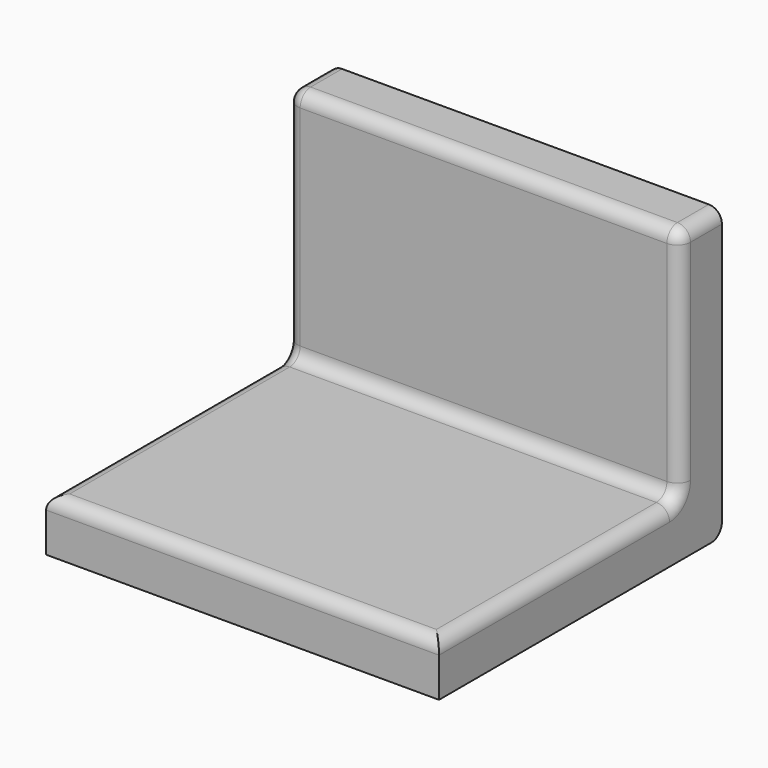
from build123d import *

# Parameters (mm, degrees)
F0_W    = 300
F0_H    = 40
F3_F1_R = 10
F3_F2_R = 10


with BuildPart() as f2:
    # F2: sweep along a path in F1
    with BuildLine(Plane.YZ) as f2_path:
        Line((0, 0), (250, 0))
        Line((250, 0), (250, 200))
    # F0 (on Front) → F2 (sweep)
    with BuildSketch(Plane.XZ):
        with Locations((4.6769320033, 0)):
            Rectangle(F0_W, F0_H)
    sweep(path=f2_path.line, transition=Transition.RIGHT)

    # F3: fillet of radius 10 on 8 edges, made by hand

    # F3_f1
    f3_f1_edges = [f2.edges().sort_by_distance(p)[0] for p in [
        (4.6769320033, 230, 20),
    ]]
    fillet(f3_f1_edges, radius=F3_F1_R)

    # F3_f2
    f3_f2_edges = [f2.edges().sort_by_distance(p)[0] for p in [
        (154.6769320033, 250, 200),
        (-145.3230679967, 250, 200),
        (154.6769320033, 110, 20),
        (4.6769320033, 0, 20),
        (-145.3230679967, 110, 20),
        (4.6769320033, 270, -20),
        (4.6769320033, 230, 200),
        (-145.3230679967, 227.0710678119, 22.9289321881),
        (154.6769320033, 227.0710678119, 22.9289321881),
    ]]
    fillet(f3_f2_edges, radius=F3_F2_R)


solid = f2.part
